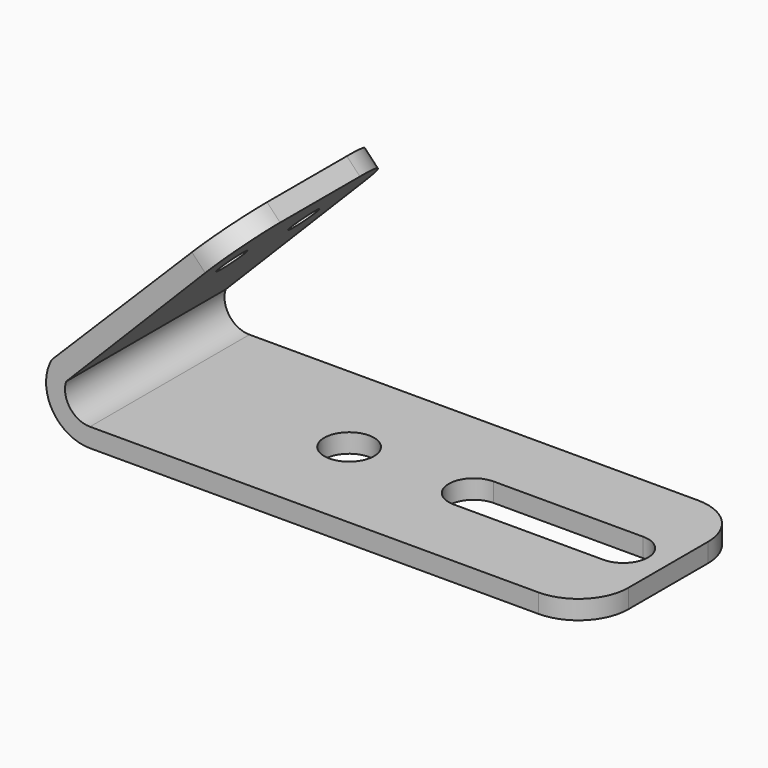
from build123d import *

# Parameters (mm, degrees)
F1_DEPTH = 254
F2_R     = 63.5
F3_DEPTH = 48.261
F4_R     = 38.1
F5_DEPTH = 49.6377001669
F6_R     = 127
F7_R     = 127


# Not quite as in the source:
# - a pattern or mirror of a feature is missing from the dataset's text; its kind, count and spacing are read off the source's solid


with BuildPart() as f1:
    # F0 (on Front) → F1 (new body, symmetric)
    with BuildSketch(Plane.XZ):
        with BuildLine():
            Line((1270, -63.5), (0, -63.5))
            ThreePointArc((0, -63.5), (-50.8447137485, -38.0403086717), (-60.9180663091, 17.9231469658))
            Line((-60.9180663091, 17.9231469658), (383.0492185975, 467.3498327088))
            Line((383.0492185975, 467.3498327088), (349.7351963182, 502.2669276563))
            Line((349.7351963182, 502.2669276563), (-96.9701293302, 55.5616020078))
            ThreePointArc((-96.9701293302, 55.5616020078), (-96.6950418594, -56.0389728653), (0, -111.76))
            Line((0, -111.76), (1270, -111.76))
            Line((1270, -111.76), (1270, -63.5))
        make_face()
    extrude(amount=F1_DEPTH, both=True)

    # F2 (on face) → F3 (cut, through all)
    with BuildSketch(Plane.XY.offset(-63.5)):
        with BuildLine():
            ThreePointArc((1155.7, -63.5), (1200.6012806053, -44.9012806053), (1219.2, 0))
            ThreePointArc((1219.2, 0), (1200.6012806053, 44.9012806053), (1155.7, 63.5))
            ThreePointArc((1155.7, 63.5), (1092.2, 0), (1155.7, -63.5))
        make_face()
        with BuildLine():
            ThreePointArc((1155.7, -63.5), (1092.2, 0), (1155.7, 63.5))
            Line((1155.7, 63.5), (774.7, 63.5))
            ThreePointArc((774.7, 63.5), (819.6012806053, 44.9012806053), (838.2, 0))
            ThreePointArc((838.2, 0), (819.6012806053, -44.9012806053), (774.7, -63.5))
            Line((774.7, -63.5), (1155.7, -63.5))
        make_face()
        with BuildLine():
            ThreePointArc((838.2, 0), (819.6012806053, 44.9012806053), (774.7, 63.5))
            ThreePointArc((774.7, 63.5), (711.2, 0), (774.7, -63.5))
            ThreePointArc((774.7, -63.5), (819.6012806053, -44.9012806053), (838.2, 0))
        make_face()
        with Locations((457.2, 0)):
            Circle(F2_R)
    extrude(amount=-F3_DEPTH, mode=Mode.SUBTRACT)

    # F4 (on face) → F5 (cut, through all)
    with BuildSketch(Plane(origin=(-76.265865669, 0, 76.265865669), x_dir=(0, -1, 0), z_dir=(-0.7071067812, 0, 0.7071067812))):
        with Locations((114.3, 411.9564794477)):
            Circle(F4_R)
    f5 = extrude(amount=-F5_DEPTH, mode=Mode.SUBTRACT)

    # F5_copies: F5 across plane
    add(f5.mirror(Plane.ZX.offset(-1e-06)), mode=Mode.SUBTRACT)

    # F6
    f6_edges = [f1.edges().sort_by_distance(p)[0] for p in [
        (366.392207, 254, 484.80838),
        (366.392207, -254, 484.80838),
    ]]
    fillet(f6_edges, radius=F6_R)

    # F7
    f7_edges = [f1.edges().sort_by_distance(p)[0] for p in [
        (1270, 254, -87.63),
        (1270, -254, -87.63),
    ]]
    fillet(f7_edges, radius=F7_R)


solid = f1.part
